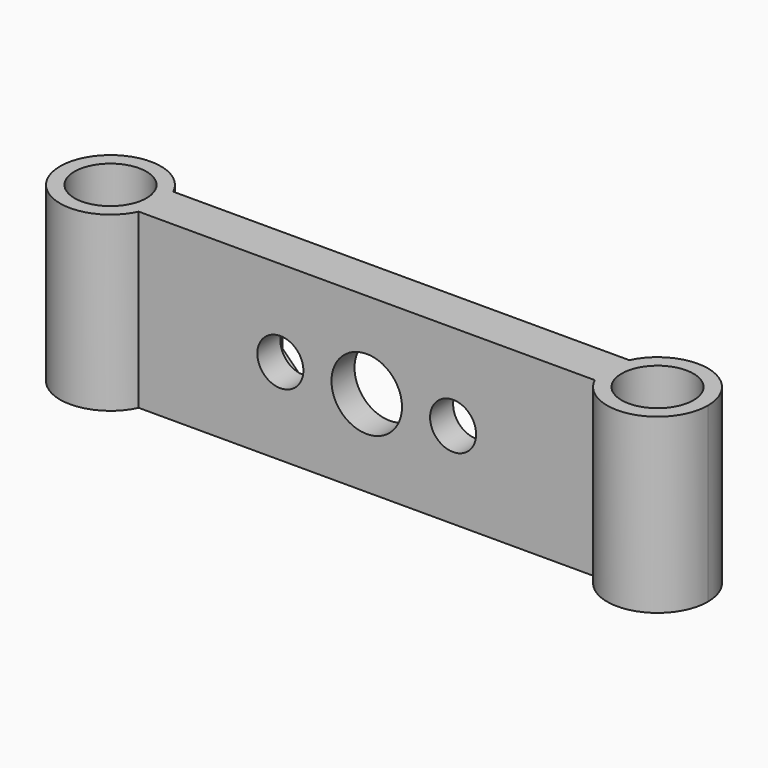
from build123d import *

# Parameters (mm, degrees)
F1_DEPTH = 12
F2_D     = 5
F2_DEPTH = 15
F2_TIP   = 1.5021515476
F3_D     = 5
F3_DEPTH = 15
F3_TIP   = 1.5021515476
F5_D     = 4.9
F5_DEPTH = 10
F5_TIP   = 1.4721085166
F6_D     = 3.2
F6_DEPTH = 15
F6_TIP   = 0.9613769904
F7_D     = 3.2
F7_DEPTH = 15
F7_TIP   = 0.9613769904
F8_W     = 16.5
F8_H     = 6.25
F9_DEPTH = 1
F10_SIZE = 2


# Not quite as in the source:
# - a feature names something its author has since deleted; it is built from what else it names


with BuildPart() as f1:
    # F0 (on Top) → F1 (new body)
    with BuildSketch(Plane.XY):
        with BuildLine():
            Line((-19, -1.8754155822), (-19, 1.1245844178))
            Line((-19, 1.1245844178), (-15.8377223398, 1.1245844178))
            ThreePointArc((-15.8377223398, 1.1245844178), (-22.5, -0.3754155822), (-15.8377223398, -1.8754155822))
            Line((-15.8377223398, -1.8754155822), (-19, -1.8754155822))
        make_face()
        with BuildLine():
            Line((-15.8377223398, 1.1245844178), (-19, 1.1245844178))
            Line((-19, 1.1245844178), (-19, -1.8754155822))
            Line((-19, -1.8754155822), (-15.8377223398, -1.8754155822))
            ThreePointArc((-15.8377223398, -1.8754155822), (-15.5854742781, -1.144189993), (-15.5, -0.3754155822))
            ThreePointArc((-15.5, -0.3754155822), (-15.5854742781, 0.3933588286), (-15.8377223398, 1.1245844178))
        make_face()
        with BuildLine():
            Line((15.8377223398, 1.1245844178), (-15.8377223398, 1.1245844178))
            ThreePointArc((-15.8377223398, 1.1245844178), (-15.5854742781, 0.3933588286), (-15.5, -0.3754155822))
            ThreePointArc((-15.5, -0.3754155822), (-15.5854742781, -1.144189993), (-15.8377223398, -1.8754155822))
            Line((-15.8377223398, -1.8754155822), (15.8377223398, -1.8754155822))
            ThreePointArc((15.8377223398, -1.8754155822), (15.5, -0.3754155822), (15.8377223398, 1.1245844178))
        make_face()
        with BuildLine():
            ThreePointArc((22.5, -0.3754155822), (19.7687744108, 3.0391101397), (15.8377223398, 1.1245844178))
            Line((15.8377223398, 1.1245844178), (19, 1.1245844178))
            Line((19, 1.1245844178), (19, -1.8754155822))
            Line((19, -1.8754155822), (15.8377223398, -1.8754155822))
            ThreePointArc((15.8377223398, -1.8754155822), (19.7687744108, -3.7899413041), (22.5, -0.3754155822))
        make_face()
        with BuildLine():
            Line((19, 1.1245844178), (15.8377223398, 1.1245844178))
            ThreePointArc((15.8377223398, 1.1245844178), (15.5, -0.3754155822), (15.8377223398, -1.8754155822))
            Line((15.8377223398, -1.8754155822), (19, -1.8754155822))
            Line((19, -1.8754155822), (19, 1.1245844178))
        make_face()
    extrude(amount=F1_DEPTH)

    # F2
    with Locations(Plane(origin=(0, 0, 0), x_dir=(1, 0, 0), z_dir=(0, 0, -1))):
        with Locations((19, 0.3754155822)):
            Hole(F2_D / 2, depth=F2_DEPTH)
            with Locations((0, 0, -(F2_DEPTH + F2_TIP / 2))):  # 118° drill point
                Cone(0, F2_D / 2, F2_TIP, mode=Mode.SUBTRACT)

    # F3
    with Locations(Plane(origin=(0, 0, 0), x_dir=(1, 0, 0), z_dir=(0, 0, -1))):
        with Locations((-19, 0.3754155822)):
            Hole(F3_D / 2, depth=F3_DEPTH)
            with Locations((0, 0, -(F3_DEPTH + F3_TIP / 2))):  # 118° drill point
                Cone(0, F3_D / 2, F3_TIP, mode=Mode.SUBTRACT)

    # F5
    with Locations(Plane(origin=(0, 1.1245844178, 0), x_dir=(-1, 0, 0), z_dir=(0, 1, 0))):
        with Locations((0, 6)):
            Hole(F5_D / 2, depth=F5_DEPTH)
            with Locations((0, 0, -(F5_DEPTH + F5_TIP / 2))):  # 118° drill point
                Cone(0, F5_D / 2, F5_TIP, mode=Mode.SUBTRACT)

    # F6
    with Locations(Plane(origin=(0, 1.1245844178, 0), x_dir=(-1, 0, 0), z_dir=(0, 1, 0))):
        with Locations((-6, 6)):
            Hole(F6_D / 2, depth=F6_DEPTH)
            with Locations((0, 0, -(F6_DEPTH + F6_TIP / 2))):  # 118° drill point
                Cone(0, F6_D / 2, F6_TIP, mode=Mode.SUBTRACT)

    # F7
    with Locations(Plane(origin=(0, 1.1245844178, 0), x_dir=(-1, 0, 0), z_dir=(0, 1, 0))):
        with Locations((6, 6)):
            Hole(F7_D / 2, depth=F7_DEPTH)
            with Locations((0, 0, -(F7_DEPTH + F7_TIP / 2))):  # 118° drill point
                Cone(0, F7_D / 2, F7_TIP, mode=Mode.SUBTRACT)

    # F8 (on face) → F9 (cut)
    with BuildSketch(Plane(origin=(0, 1.1245844178, 0), x_dir=(-1, 0, 0), z_dir=(0, 1, 0))):
        with Locations((0, 6)):
            Rectangle(F8_W, F8_H)
    extrude(amount=-F9_DEPTH, mode=Mode.SUBTRACT)

    # F10
    f10_edges = [f1.edges().sort_by_distance(p)[0] for p in [
        (8.25, 0.624584, 9.125),
        (8.25, 0.624584, 2.875),
        (-8.25, 0.624584, 9.125),
        (-8.25, 0.624584, 2.875),
    ]]
    chamfer(f10_edges, length=F10_SIZE)


solid = f1.part
